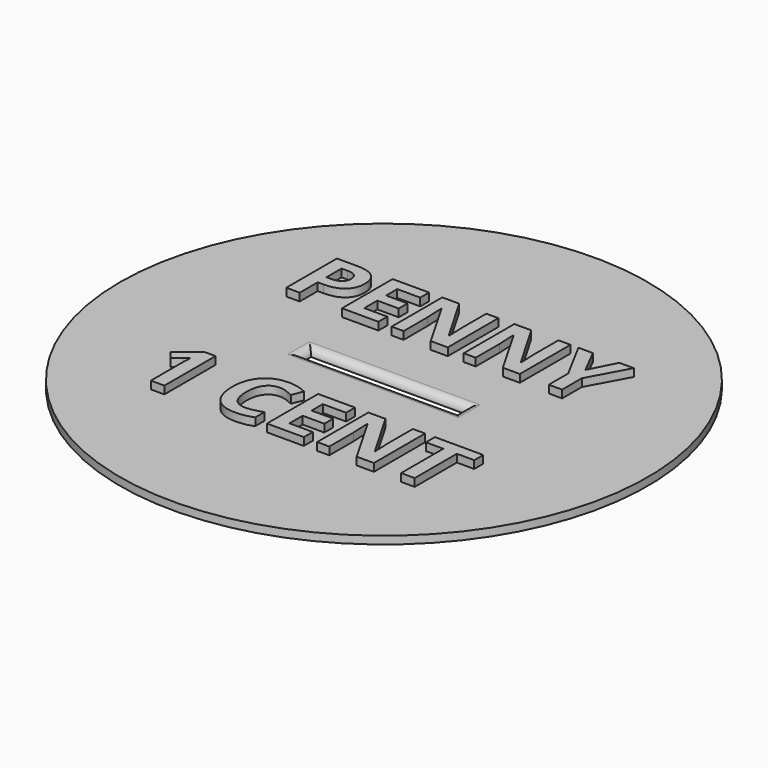
from build123d import *

# Parameters (mm, degrees)
F0_W           = 34
F0_H           = 1
F2_W           = 20
F2_H           = 1.52
F3_DEPTH       = 1.001
F4_R           = 0.99999
F5_TEXT_SIZE   = 11.4193951289
F5_TEXT_SIZE_2 = 11.5450527645
F6_DEPTH       = 1


# Not quite as in the source:
# - a fillet or chamfer is up to 0.001 mm smaller than in the source, because OpenCascade refuses the exact size
# - Text() gives the source's letters only with a copy of the font that has no kerning and outlines rounded to 1/6400 em; it was checked with that copy


with BuildPart() as f1:
    # F0 (on Front) → F1 (revolve)
    with BuildSketch(Plane.XZ):
        with Locations((-17, 0.5)):
            Rectangle(F0_W, F0_H)
    revolve(axis=Axis((0, 0, 0.5), (0, 0, 1)))

    # F2 (on Top) → F3 (cut, through all)
    with BuildSketch(Plane.XY):
        Rectangle(F2_W, F2_H)
    extrude(amount=F3_DEPTH, mode=Mode.SUBTRACT)

    # F4 (radius 1 in the source; OpenCascade refuses exactly that, so slightly less here)
    f4_edges = [f1.edges().sort_by_distance(p)[0] for p in [
        (0, 0.76, 1),
        (-10, 0, 1),
        (0, -0.76, 1),
        (10, 0, 1),
    ]]
    fillet(f4_edges, radius=F4_R)

    # F5 (on face) → F6 (join)
    with BuildSketch(Plane.XY.offset(1)):
        with Locations((-20, 8)):
            Text('PENNY', F5_TEXT_SIZE, font='Open Sans', font_style=FontStyle.BOLD, text_align=(TextAlign.LEFT, TextAlign.BOTTOM))
        with Locations((-20, -16.3124379904)):
            Text('1 CENT', F5_TEXT_SIZE_2, font='Open Sans', font_style=FontStyle.BOLD, text_align=(TextAlign.LEFT, TextAlign.BOTTOM))
    extrude(amount=F6_DEPTH)


solid = f1.part
